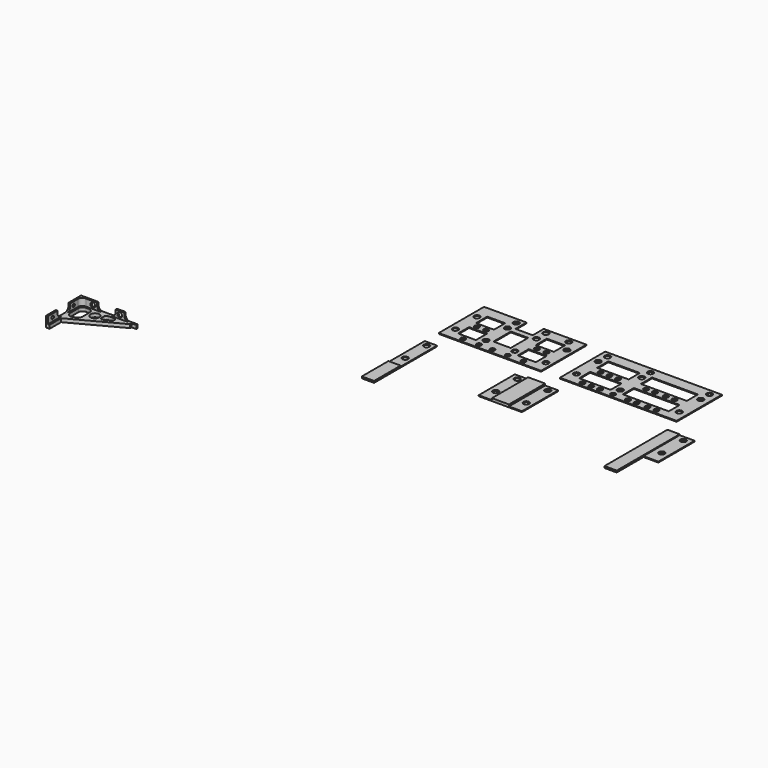
from build123d import *

# Parameters (mm, degrees)
F0_R      = 3.25
F0_W      = 20.75
F0_H      = 10
F0_R_2    = 2.75
F0_W_2    = 19.75
F0_H_2    = 7.5
F0_H_3    = 6.5000051176
F0_W_3    = 20.5
F1_DEPTH  = 1
F0_W_4    = 52.4999990344
F0_W_5    = 36
F0_W_6    = 14
F0_H_4    = 38.25
F0_H_5    = 51.75
F0_W_7    = 15
F0_W_8    = 19.5
F0_W_9    = 17
F2_W      = 14
F2_H      = 37.9871611556
F5_DEPTH  = 1
F6_DEPTH  = 1
F3_W      = 19.5
F3_H      = 51.75
F7_DEPTH  = 2
F0_R_3    = 5
F8_DEPTH  = 4
F9_W      = 18
F9_H      = 2
F9_W_2    = 10
F9_W_3    = 2
F9_H_2    = 14
F10_DEPTH = 8
F11_R     = 1.75
F12_DEPTH = 4
F13_R     = 2.75
F14_DEPTH = 2
F15_R     = 5
F16_R     = 2.5


# Not quite as in the source:
# - a feature names something its author has since deleted; it is built from what else it names


with BuildPart() as f1:
    # F0 (on Top) → F1 (new body)
    with BuildSketch(Plane.XY):
        Polygon((-171.6413756013, 28.2858474609), (-206.1413746923, 28.2858498732), (-206.1413756013, 15.2858447556), (-192.1413756013, 15.2858447556), (-171.6413756013, 15.2858447556), align=None)
        Polygon((-103.1413756013, 15.2858413724), (-89.1413748748, 15.2858403935), (-89.1413746923, 28.2858370699), (-123.8913756013, 28.2858394996), (-123.8913756013, 15.2858428233), align=None)
        with Locations((-104.6413751468, 22.5877612829)):
            Circle(F0_R, mode=Mode.SUBTRACT)
        with Locations((-113.5163756013, -5.7141552444)):
            Rectangle(F0_W, F0_H)
        with Locations((-118.4663661122, -5.7141552444)):
            Circle(F0_R_2, mode=Mode.SUBTRACT)
        with Locations((-107.7163661122, -5.7141552444)):
            Circle(F0_R_2, mode=Mode.SUBTRACT)
        Polygon((-192.1413756013, -26.4641539697), (-192.1413756013, -36.4641501268), (-103.1413756013, -36.4641501268), (-103.1413756013, -26.4641539697), (-123.8913756013, -26.4641539697), (-137.8913756013, -26.4641539697), (-157.6413756013, -26.4641539697), (-171.6413756013, -26.4641539697), align=None)
        with Locations((-182.1413756013, -31.6281057894)):
            Circle(F0_R_2, mode=Mode.SUBTRACT)
        with Locations((-164.1413751468, -31.6281057894)):
            Circle(F0_R_2, mode=Mode.SUBTRACT)
        with Locations((-148.694768548, -31.6281501268)):
            Circle(F0_R_2, mode=Mode.SUBTRACT)
        with Locations((-131.1413751468, -31.6281057894)):
            Circle(F0_R_2, mode=Mode.SUBTRACT)
        with Locations((-113.1413756013, -31.6281501268)):
            Circle(F0_R_2, mode=Mode.SUBTRACT)
        with Locations((-147.7663756013, -22.7141539697)):
            Rectangle(F0_W_2, F0_H_2)
        with Locations((-147.7663756013, 9.2858434715)):
            Rectangle(F0_W_2, F0_H_3)
        with Locations((-181.8913756013, -5.7141552444)):
            Rectangle(F0_W_3, F0_H)
        with Locations((-187.1413756013, -5.7141539697)):
            Circle(F0_R_2, mode=Mode.SUBTRACT)
        with Locations((-176.6413756013, -5.7141539697)):
            Circle(F0_R_2, mode=Mode.SUBTRACT)
        Polygon((-157.6413756013, 15.2858447556), (-171.6413756013, 15.2858447556), (-171.6413756013, -0.7141552444), (-171.6413756013, -10.7141552444), (-171.6413756013, -26.4641539697), (-157.6413756013, -26.4641539697), (-157.6413756013, -18.9641539697), (-157.6413756013, 6.0358409127), (-157.6413756013, 12.5358460303), align=None)
        with Locations((-164.1413751468, -21.4641539697)):
            Circle(F0_R, mode=Mode.SUBTRACT)
        with Locations((-164.1413751468, 9.2858409127)):
            Circle(F0_R, mode=Mode.SUBTRACT)
        Polygon((-157.6413756013, 28.285846482), (-171.6413756013, 28.2858474609), (-171.6413756013, 15.2858447556), (-157.6413756013, 15.2858447556), align=None)
        with Locations((-164.1413751468, 21.7858469365)):
            Circle(F0_R, mode=Mode.SUBTRACT)
        Polygon((-137.8913756013, 28.2858404785), (-137.8913756013, 15.2858438022), (-123.8913756013, 15.2858428233), (-123.8913756013, 28.2858394996), align=None)
        with Locations((-131.1413751468, 22.7858400066)):
            Circle(F0_R, mode=Mode.SUBTRACT)
        Polygon((-137.8913756013, 15.2858438022), (-137.8913756013, 12.5358460303), (-137.8913756013, 6.0358409127), (-137.8913756013, -18.9641539697), (-137.8913756013, -26.4641539697), (-123.8913756013, -26.4641539697), (-123.8913756013, -10.7141552444), (-123.8913756013, -0.7141552444), (-123.8913756013, 15.2858428233), align=None)
        with Locations((-131.1413751468, -21.4641539697)):
            Circle(F0_R, mode=Mode.SUBTRACT)
        with Locations((-131.1413751468, 9.2858409127)):
            Circle(F0_R, mode=Mode.SUBTRACT)
        Polygon((-103.1413756013, -26.4641539697), (-103.1413756013, -36.4641501268), (-89.1413756013, -36.4641501268), (-89.1413748748, 15.2858403935), (-103.1413756013, 15.2858413724), (-103.1413756013, -0.7141552444), (-103.1413756013, -10.7141552444), align=None)
        with Locations((-95.6413756013, -21.4641539697)):
            Circle(F0_R, mode=Mode.SUBTRACT)
        with Locations((-96.1413751908, 9.2858409127)):
            Circle(F0_R, mode=Mode.SUBTRACT)
        Polygon((-192.1413756013, 15.2858447556), (-206.1413756013, 15.2858447556), (-206.1413756013, -36.4641501268), (-192.1413756013, -36.4641501268), (-192.1413756013, -26.4641539697), (-192.1413756013, -10.7141552444), (-192.1413756013, -0.7141552444), align=None)
        with Locations((-199.1413756013, -21.4641539697)):
            Circle(F0_R, mode=Mode.SUBTRACT)
        with Locations((-199.1413756013, 9.2858409127)):
            Circle(F0_R, mode=Mode.SUBTRACT)
    extrude(amount=F1_DEPTH)


with BuildPart() as f1b:
    # F0 (on Top) → F1, piece 2 (new body)
    with BuildSketch(Plane.XY):
        Polygon((65.8586253077, 28.2858370699), (-67.6413746923, 28.2858370699), (-67.6413756013, 15.2858447556), (-53.6413756013, 15.2858370699), (-17.6413756013, 15.2858370699), (-3.6413756013, 15.2858370699), (48.8586234331, 15.2858370699), (65.8586243987, 15.2858370699), align=None)
        with Locations((-59.6413751468, 21.7858447556)):
            Circle(F0_R, mode=Mode.SUBTRACT)
        with Locations((-10.6413751468, 21.7858447556)):
            Circle(F0_R, mode=Mode.SUBTRACT)
        with Locations((56.8586248532, 21.7858447556)):
            Circle(F0_R, mode=Mode.SUBTRACT)
        with Locations((22.6086239159, -5.7141552444)):
            Rectangle(F0_W_4, F0_H)
        with Locations((6.3586243987, -5.7141552444)):
            Circle(F0_R_2, mode=Mode.SUBTRACT)
        with Locations((16.3586243987, -5.7141552444)):
            Circle(F0_R_2, mode=Mode.SUBTRACT)
        with Locations((28.8586234331, -5.7141552444)):
            Circle(F0_R_2, mode=Mode.SUBTRACT)
        with Locations((38.8586234331, -5.7141552444)):
            Circle(F0_R_2, mode=Mode.SUBTRACT)
        Polygon((-53.6413756013, -26.4641552444), (-53.6413756013, -36.4641501268), (48.8586243987, -36.4641501268), (48.8586234331, -26.4641501751), (-3.6413756013, -26.4641552444), (-17.6413756013, -26.4641552444), align=None)
        with Locations((-45.6413756013, -31.6281501268)):
            Circle(F0_R_2, mode=Mode.SUBTRACT)
        with Locations((-35.6413756013, -31.6281501268)):
            Circle(F0_R_2, mode=Mode.SUBTRACT)
        with Locations((-25.6413756013, -31.6281501268)):
            Circle(F0_R_2, mode=Mode.SUBTRACT)
        with Locations((-10.6413756013, -31.6281501268)):
            Circle(F0_R_2, mode=Mode.SUBTRACT)
        with Locations((6.3586243987, -31.6281501268)):
            Circle(F0_R_2, mode=Mode.SUBTRACT)
        with Locations((16.3586243987, -31.6281501268)):
            Circle(F0_R_2, mode=Mode.SUBTRACT)
        with Locations((28.8586234331, -31.6281501268)):
            Circle(F0_R_2, mode=Mode.SUBTRACT)
        with Locations((38.8586234331, -31.6281501268)):
            Circle(F0_R_2, mode=Mode.SUBTRACT)
        Polygon((-3.6413756013, 15.2858370699), (-17.6413756013, 15.2858370699), (-17.6413756013, -0.7141552444), (-17.6413756013, -10.7141552444), (-17.6413756013, -26.4641552444), (-3.6413756013, -26.4641552444), (-3.6413756013, -10.7141552444), (-3.6413756013, -0.7141552444), align=None)
        with Locations((-10.6413751468, -21.4641539697)):
            Circle(F0_R, mode=Mode.SUBTRACT)
        with Locations((-10.6413751468, 9.2858409127)):
            Circle(F0_R, mode=Mode.SUBTRACT)
        with Locations((-35.6413756013, -5.7141552444)):
            Rectangle(F0_W_5, F0_H)
        with Locations((-45.6413756013, -5.7141552444)):
            Circle(F0_R_2, mode=Mode.SUBTRACT)
        with Locations((-35.6413756013, -5.7141552444)):
            Circle(F0_R_2, mode=Mode.SUBTRACT)
        with Locations((-25.6413756013, -5.7141552444)):
            Circle(F0_R_2, mode=Mode.SUBTRACT)
        Polygon((65.8586243987, -36.4641501268), (65.8586243987, 15.2858370699), (48.8586234331, 15.2858370699), (48.8586234331, -0.7141552444), (48.8586234331, -10.7141552444), (48.8586234331, -26.4641501751), (48.8586243987, -36.4641501268), align=None)
        with Locations((56.8586248532, -21.4641501268)):
            Circle(F0_R, mode=Mode.SUBTRACT)
        with Locations((56.8586248532, 9.2858409127)):
            Circle(F0_R, mode=Mode.SUBTRACT)
        Polygon((-53.6413756013, 15.2858370699), (-67.6413756013, 15.2858447556), (-67.6413756013, -36.4641501268), (-53.6413756013, -36.4641501268), (-53.6413756013, -26.4641552444), (-53.6413756013, -10.7141552444), (-53.6413756013, -0.7141552444), align=None)
        with Locations((-60.6413756013, -21.4641539697)):
            Circle(F0_R, mode=Mode.SUBTRACT)
        with Locations((-60.6413756013, 9.2858409127)):
            Circle(F0_R, mode=Mode.SUBTRACT)
    extrude(amount=F1_DEPTH)


with BuildPart() as f1c:
    # F0 (on Top) → F1, piece 3 (new body)
    with BuildSketch(Plane.XY):
        with Locations((-199.1413756013, -127.3391501268)):
            Rectangle(F0_W_6, F0_H_4)
        with Locations((-199.1413756013, -82.3391501268)):
            Rectangle(F0_W_6, F0_H_5)
        with Locations((-199.1413756013, -93.2141501268)):
            Circle(F0_R, mode=Mode.SUBTRACT)
        with Locations((-199.1413756013, -62.4641501268)):
            Circle(F0_R, mode=Mode.SUBTRACT)
    extrude(amount=F1_DEPTH)

    # F2 (on face) → F5 (join)
    with BuildSketch(Plane.XY.offset(1)):
        with Locations((-199.1413756013, -127.470569549)):
            Rectangle(F2_W, F2_H)
    extrude(amount=F5_DEPTH)


with BuildPart() as f1d:
    # F0 (on Top) → F1, piece 4 (new body)
    with BuildSketch(Plane.XY):
        with Locations((-95.6413756013, -82.3391501268)):
            Rectangle(F0_W_7, F0_H_5)
        with Locations((-95.6413756013, -93.2181501268)):
            Circle(F0_R, mode=Mode.SUBTRACT)
        with Locations((-95.6413756013, -62.4641501268)):
            Circle(F0_R, mode=Mode.SUBTRACT)
        with Locations((-61.1413756013, -82.3391501268)):
            Rectangle(F0_W_7, F0_H_5)
        with Locations((-60.6413756013, -93.2181501268)):
            Circle(F0_R, mode=Mode.SUBTRACT)
        with Locations((-60.6413756013, -62.4641501268)):
            Circle(F0_R, mode=Mode.SUBTRACT)
        with Locations((-78.3913756013, -82.3391501268)):
            Rectangle(F0_W_8, F0_H_5)
    extrude(amount=F1_DEPTH)

    # F3 (on face) → F7 (join)
    with BuildSketch(Plane.XY.offset(1)):
        with Locations((-78.214810431, -82.3391501268)):
            Rectangle(F3_W, F3_H)
    extrude(amount=F7_DEPTH)


with BuildPart() as f1e:
    # F0 (on Top) → F1, piece 5 (new body)
    with BuildSketch(Plane.XY):
        Polygon((85.3586243987, -56.4641501268), (71.3586243987, -56.4641501268), (71.3586243987, -146.4641501268), (85.3586243987, -146.4641501268), (85.3586243987, -108.2141501268), align=None)
        with Locations((93.8586243987, -82.3391501268)):
            Rectangle(F0_W_9, F0_H_5)
        with Locations((94.3586243987, -93.2181501268)):
            Circle(F0_R, mode=Mode.SUBTRACT)
        with Locations((94.3586243987, -62.4641501268)):
            Circle(F0_R, mode=Mode.SUBTRACT)
    extrude(amount=F1_DEPTH)

    # F4 (on face) → F6 (join)
    with BuildSketch(Plane.XY.offset(1)):
        Polygon((85.3586243987, -108.2141501268), (85.3586243987, -56.4641501268), (71.3586243987, -56.4641501268), (71.3586243987, -146.4641501268), (85.3586243987, -146.4641501268), align=None)
    extrude(amount=F6_DEPTH)


with BuildPart() as f8:
    # F0 (on Top) → F8 (new body)
    with BuildSketch(Plane.XY):
        Polygon((-483.6915080496, -229.3373813054), (-428.3476592873, -199.8624135239), (-428.3476592873, -197.8624135239), (-422.9415080496, -197.8624135239), (-422.9415080496, -195.8624135239), (-487.6915080496, -195.8624135239), (-487.6915080496, -245.8624135239), (-483.6915080496, -245.8624135239), align=None)
        Polygon((-483.6915080496, -224.8054672424), (-483.6915080496, -199.8624135239), (-470.6915080496, -199.8624135239), (-456.0195836684, -199.8624135239), (-436.8570347128, -199.8624135239), (-456.0195836684, -210.0679833516), (-470.6915080496, -217.8819411464), align=None, mode=Mode.SUBTRACT)
        Polygon((-456.0195836684, -199.8624135239), (-470.6915080496, -199.8624135239), (-470.6915080496, -217.8819411464), (-456.0195836684, -210.0679833516), align=None)
        with Locations((-463.0195836684, -206.8624135239)):
            Circle(F0_R_3, mode=Mode.SUBTRACT)
    extrude(amount=F8_DEPTH)

    # F9 (on face) → F10 (join)
    with BuildSketch(Plane.XY.offset(4)):
        Polygon((-485.6915080496, -195.8624135239), (-487.6915080496, -195.8624135239), (-487.6915080496, -213.8624135239), (-485.6915080496, -213.8624135239), (-485.6915080496, -197.8624135239), align=None)
        with Locations((-476.6915080496, -196.8624135239)):
            Rectangle(F9_W, F9_H)
        with Locations((-441.6915080496, -196.8624135239)):
            Rectangle(F9_W_2, F9_H)
        with Locations((-486.6915080496, -238.8624135239)):
            Rectangle(F9_W_3, F9_H_2)
    extrude(amount=F10_DEPTH)

    # F11 (on face) → F12 (cut)
    with BuildSketch(Plane(origin=(-487.6915080496, 0, 0), x_dir=(0, -1, 0), z_dir=(-1, 0, 0))):
        with Locations((208.8624135239, 8)):
            Circle(F11_R)
        with Locations((238.8624135239, 8)):
            Circle(F11_R)
    extrude(amount=-F12_DEPTH, mode=Mode.SUBTRACT)

    # F13 (on face) → F14 (cut)
    with BuildSketch(Plane(origin=(0, -195.8624135239, 0), x_dir=(-1, 0, 0), z_dir=(0, 1, 0))):
        with Locations((441.9415080496, 8)):
            Circle(F13_R)
        with Locations((472.6915080496, 8)):
            Circle(F13_R)
    extrude(amount=-F14_DEPTH, mode=Mode.SUBTRACT)

    # F15
    f15_edges = [f8.edges().sort_by_distance(p)[0] for p in [
        (-485.691508, -197.862414, 8),
        (-467.691508, -196.862414, 4),
        (-436.691508, -196.862414, 4),
        (-446.691508, -196.862414, 4),
        (-483.691508, -199.862414, 2),
        (-470.691508, -199.862414, 2),
        (-470.691508, -217.881941, 2),
        (-483.691508, -224.805467, 2),
        (-486.691508, -213.862414, 4),
        (-486.691508, -231.862414, 4),
    ]]
    fillet(f15_edges, radius=F15_R)

    # F16
    f16_edges = [f8.edges().sort_by_distance(p)[0] for p in [
        (-456.019584, -199.862414, 2),
        (-456.019584, -210.067983, 2),
        (-436.857035, -199.862414, 2),
    ]]
    fillet(f16_edges, radius=F16_R)


solid = Compound([f1.part, f1b.part, f1c.part, f1d.part, f1e.part, f8.part])
